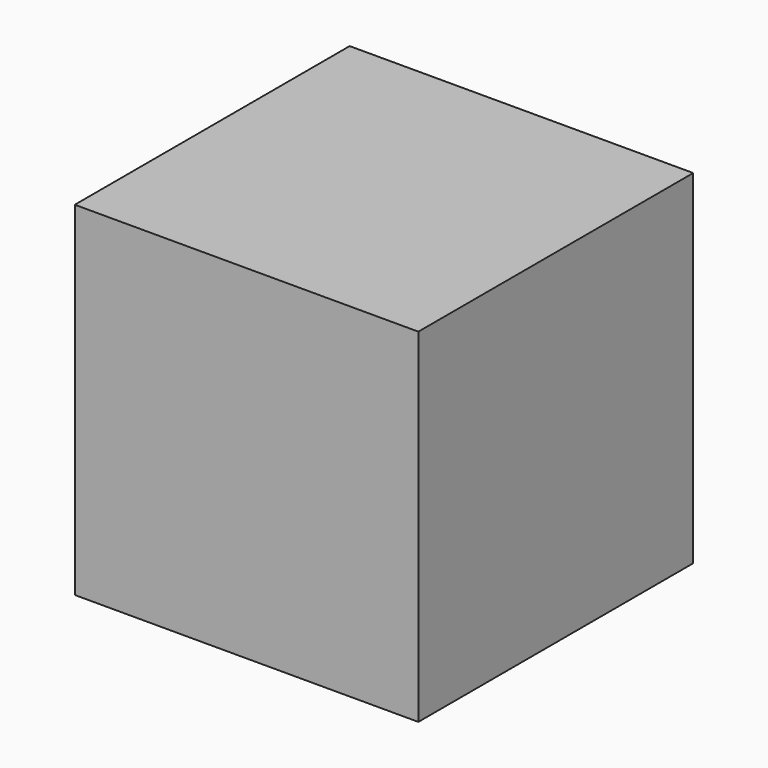
from build123d import *

# Parameters (mm, degrees)
F1_W     = 101.6
F1_H     = 101.6
F2_DEPTH = 50.8
F3_W     = 38.1
F3_H     = 38.1
F4_DEPTH = 25.4
F5_DEPTH = 25.4


# Not quite as in the source:
# - a variable given as a bare number and used for a length is read in inches; the dataset says mm whatever the document's units were


with BuildPart() as f2:
    # F1 (on Front) → F2 (new body, symmetric)
    with BuildSketch(Plane.XZ):
        Rectangle(F1_W, F1_H)
    extrude(amount=F2_DEPTH, both=True)

    # F3 (on face) → F4 (join)
    with BuildSketch(Plane.XZ.offset(50.8)):
        Rectangle(F3_W, F3_H)
    extrude(amount=F4_DEPTH)

    # F5 (cut): a face of the model
    f5_faces = [f2.faces().sort_by_distance(p)[0] for p in [
        (0, -76.2, 0),
    ]]
    extrude(f5_faces, amount=-F5_DEPTH, mode=Mode.SUBTRACT)


solid = f2.part
